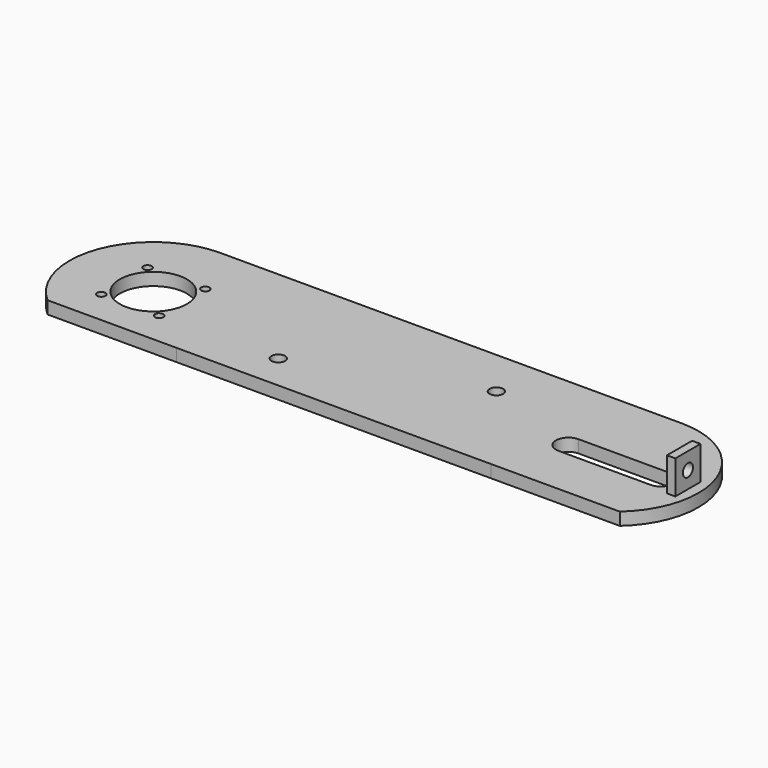
from build123d import *

# Parameters (mm, degrees)
F0_R     = 3.25
F0_R_2   = 16
F1_DEPTH = 6
F2_W     = 4
F2_H     = 15
F3_DEPTH = 16
F4_R     = 3
F5_DEPTH = 25
F6_R     = 2
F6_R_2   = 16
F7_DEPTH = 25


# Not quite as in the source:
# - ends of sketch curves that miss each other by under 0.0002 mm in the source are joined


with BuildPart() as f1:
    # F0 (on Top) → F1 (new body)
    with BuildSketch(Plane.XY):
        with BuildLine():
            ThreePointArc((136.4575130484, -35.0000000549), (147.4165738824, 9.1421355849), (110, 35))
            Line((110, 35), (75, 35))
            Line((75, 35), (-75, 35))
            Line((-75, 35), (-110, 35))
            ThreePointArc((-110, 35), (-147.4165737498, 9.1421359357), (-136.4575136109, -34.9999995588))
            Line((-136.4575136109, -34.9999995588), (-75, -35))
            Line((-75, -35), (75, -35))
            Line((75, -35), (136.4575130484, -35.0000000549))
        make_face()
        with Locations((-40, -18)):
            Circle(F0_R, mode=Mode.SUBTRACT)
        with Locations((-110, -5)):
            Circle(F0_R_2, mode=Mode.SUBTRACT)
        with BuildLine():
            Line((88, 1), (132, 1))
            ThreePointArc((132, 1), (137.9996084013, -5.0685494815), (131.862909985, -10.9984336562))
            Line((131.862909985, -10.9984336562), (88.000112, -11))
            ThreePointArc((88.000112, -11), (82.0000000003, -5.000056), (88, 1))
        make_face(mode=Mode.SUBTRACT)
        with Locations((40, 12)):
            Circle(F0_R, mode=Mode.SUBTRACT)
    extrude(amount=F1_DEPTH)

    # F2 (on face) → F3 (join)
    with BuildSketch(Plane.XY.offset(6)):
        with Locations((143, -5.0685494815)):
            Rectangle(F2_W, F2_H)
    extrude(amount=F3_DEPTH)

    # F4 (on face) → F5 (cut)
    with BuildSketch(Plane.YZ.offset(145)):
        with Locations((-5.0685494815, 14)):
            Circle(F4_R)
    extrude(amount=-F5_DEPTH, mode=Mode.SUBTRACT)

    # F6 (on face) → F7 (cut)
    with BuildSketch(Plane.XY.offset(6)):
        with Locations((-123.7885822331, 8.7885822331)):
            Circle(F6_R)
        with Locations((-96.2114177669, 8.7885822331)):
            Circle(F6_R)
        with Locations((-96.2114177669, -18.7885822331)):
            Circle(F6_R)
        with Locations((-123.7885822331, -18.7885822331)):
            Circle(F6_R)
        with Locations((-110, -5)):
            Circle(F6_R_2)
    extrude(amount=-F7_DEPTH, mode=Mode.SUBTRACT)


solid = f1.part
